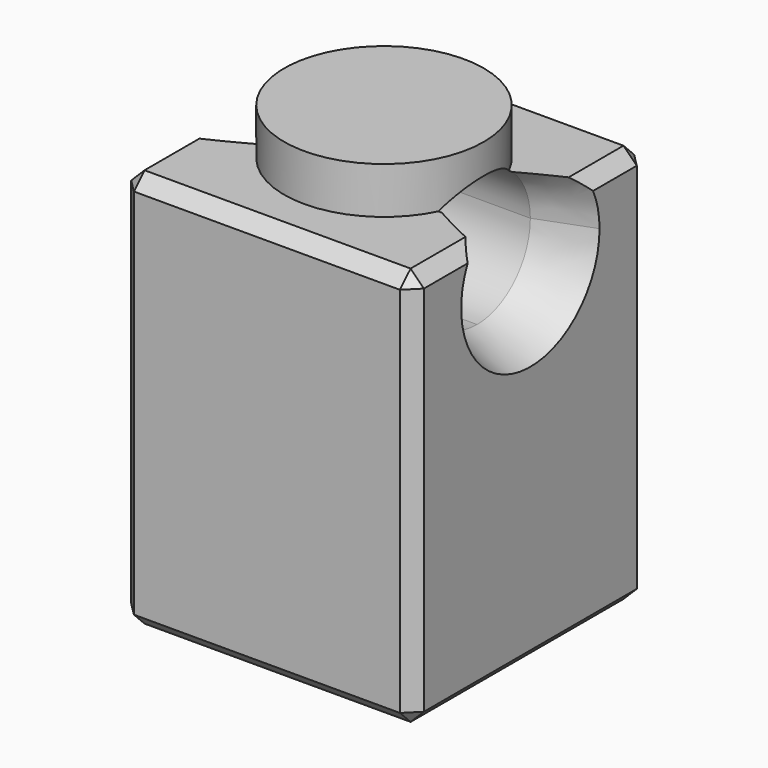
from build123d import *

# Parameters (mm, degrees)
F2_W          = 44
F2_H          = 44
F2_R          = 15
F2_R_2        = 10
F3_DEPTH      = 60
F4_R          = 15
F4_R_2        = 10
F5_DEPTH      = 7
F6_DEPTH      = 9
F8_SIZE       = 2
F11_DEPTH     = 60
F12_T4_ANGLE  = 332.4696617
F12_T9_ANGLE  = 152.2075678766
F12_T14_ANGLE = 152.2075678766
F12_T19_ANGLE = 332.4696617


# Not quite as in the source:
# - a fillet or chamfer that OpenCascade refuses, or shapes differently, is made with other operations: its cross-section is extruded or revolved along the edge and cut away or added


with BuildPart() as f3:
    # F2 (on Top) → F3 (new body)
    with BuildSketch(Plane.XY):
        Rectangle(F2_W, F2_H)
        Circle(F2_R, mode=Mode.SUBTRACT)
        Circle(F2_R)
        Circle(F2_R_2, mode=Mode.SUBTRACT)
        Circle(F2_R_2)
    extrude(amount=F3_DEPTH)

    # F4 (on face) → F5 (join)
    with BuildSketch(Plane.XY.offset(60)):
        Circle(F4_R)
        Circle(F4_R_2, mode=Mode.SUBTRACT)
        Circle(F4_R_2)
    extrude(amount=F5_DEPTH)

    # F2 (on Top) → F6 (cut)
    with BuildSketch(Plane.XY):
        Circle(F2_R)
        Circle(F2_R_2, mode=Mode.SUBTRACT)
        Circle(F2_R_2)
    extrude(amount=F6_DEPTH, mode=Mode.SUBTRACT)

    # F8
    f8_edges = [f3.edges().sort_by_distance(p)[0] for p in [
        (0, -22, 0),
        (22, 0, 0),
        (-22, 0, 0),
        (0, 22, 0),
        (-22, -22, 30),
        (-22, 22, 30),
        (22, 22, 30),
        (22, -22, 30),
        (22, 0, 60),
        (0, -22, 60),
        (-22, 0, 60),
        (0, 22, 60),
        (-15, 0, 0),
    ]]
    chamfer(f8_edges, length=F8_SIZE)

    # F10 (on offset) → F11 (cut)
    with BuildSketch(Plane.YZ.offset(22)):
        with BuildLine():
            ThreePointArc((10, 52.5087859035), (7.0710678119, 59.5798537153), (0, 62.5087859035))
            Line((0, 62.5087859035), (0, 42.5087859035))
            ThreePointArc((0, 42.5087859035), (7.0710678119, 45.4377180916), (10, 52.5087859035))
        make_face()
        with BuildLine():
            Line((0, 42.5087859035), (0, 62.5087859035))
            ThreePointArc((0, 62.5087859035), (-10, 52.5087859035), (0, 42.5087859035))
        make_face()
    extrude(amount=-F11_DEPTH, mode=Mode.SUBTRACT)

    # F12: chamfer of 3 x 8 on 4 edges, made by hand


with BuildPart() as f12_tool2:
    # F12_s3 → F12_t4 (revolve)
    with BuildSketch(Plane(origin=(0, -21.5222750688, 41.2905103072), x_dir=(1, 0, 0), z_dir=(0, 0.4622182236, -0.8867662115))):
        Polygon((-22, -37.2705177426), (-14, -34.2705177426), (-22, -34.2705177426), align=None)
    revolve(axis=Axis((-22, 0, 52.5087859035), (1, 0, 0)), revolution_arc=F12_T4_ANGLE)

    split(bisect_by=Plane.XY.offset(60), keep=Keep.BOTTOM)


with BuildPart() as f3_1:
    add(f3.part)

    # F12_t1: cut F12_tool2
    add(f12_tool2.part, mode=Mode.SUBTRACT)


with BuildPart() as f12_tool7:
    # F12_s8 → F12_t9 (revolve)
    with BuildSketch(Plane.XY.offset(52.5087859035)):
        Polygon((-22, 13), (-14, 10), (-22, 10), align=None)
    revolve(axis=Axis((-22, 0, 52.5087859035), (1, 0, 0)), revolution_arc=F12_T9_ANGLE)

    split(bisect_by=Plane.XY.offset(60), keep=Keep.BOTTOM)


with BuildPart() as f3_2:
    add(f3_1.part)

    # F12_t6: cut F12_tool7
    add(f12_tool7.part, mode=Mode.SUBTRACT)


with BuildPart() as f12_tool12:
    # F12_s13 → F12_t14 (revolve)
    with BuildSketch(Plane.XY.offset(52.5087859035)):
        Polygon((22, 13), (14, 10), (22, 10), align=None)
    revolve(axis=Axis((22, 0, 52.5087859035), (1, 0, 0)), revolution_arc=F12_T14_ANGLE)

    split(bisect_by=Plane.XY.offset(60), keep=Keep.BOTTOM)


with BuildPart() as f3_3:
    add(f3_2.part)

    # F12_t11: cut F12_tool12
    add(f12_tool12.part, mode=Mode.SUBTRACT)


with BuildPart() as f12_tool17:
    # F12_s18 → F12_t19 (revolve)
    with BuildSketch(Plane(origin=(0, -21.5222750688, 41.2905103072), x_dir=(1, 0, 0), z_dir=(0, 0.4622182236, -0.8867662115))):
        Polygon((22, -37.2705177426), (14, -34.2705177426), (22, -34.2705177426), align=None)
    revolve(axis=Axis((22, 0, 52.5087859035), (1, 0, 0)), revolution_arc=F12_T19_ANGLE)

    split(bisect_by=Plane.XY.offset(60), keep=Keep.BOTTOM)


with BuildPart() as f3_4:
    add(f3_3.part)

    # F12_t16: cut F12_tool17
    add(f12_tool17.part, mode=Mode.SUBTRACT)


solid = f3_4.part
